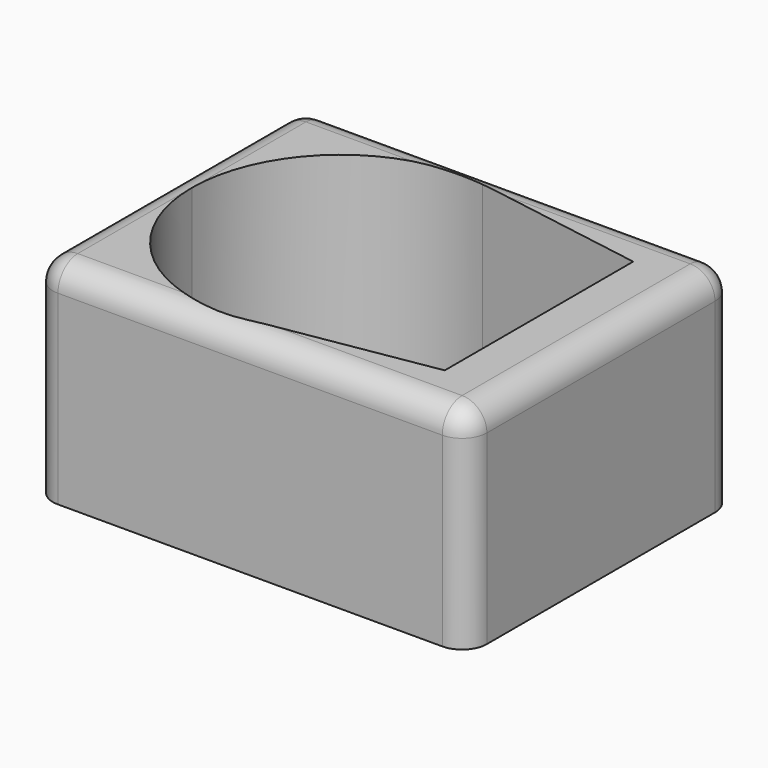
from build123d import *

# Parameters (mm, degrees)
F0_W         = 35
F0_H         = 27
F1_DEPTH     = 15
F2_DEPTH     = 2
F3_T1_DEPTH  = 20
F3_T3_DEPTH  = 31
F3_T5_DEPTH  = 23
F3_S9_W      = 2
F3_S9_H      = 2
F3_T10_DEPTH = 2
F3_S15_W     = 2
F3_S15_H     = 2
F3_T16_DEPTH = 2
F3_S21_W     = 2
F3_S21_H     = 2
F3_T22_DEPTH = 2
F3_S27_W     = 2
F3_S27_H     = 2
F3_T28_DEPTH = 2


# Not quite as in the source:
# - a fillet or chamfer that OpenCascade refuses, or shapes differently, is made with other operations: its cross-section is extruded or revolved along the edge and cut away or added


with BuildPart() as f1:
    # F0 (on Top) → F1 (new body)
    with BuildSketch(Plane.XY):
        with Locations((-13.2022674233, 7.6325895488)):
            Rectangle(F0_W, F0_H)
        with BuildLine():
            Line((-14.73041686, 19.4694728107), (-0.7022674233, 17.1325895488))
            Line((-0.7022674233, 17.1325895488), (-0.7022674233, 7.6325895488))
            Line((-0.7022674233, 7.6325895488), (-0.7022674233, -1.8674104512))
            Line((-0.7022674233, -1.8674104512), (-14.73041686, -4.2042937131))
            ThreePointArc((-14.73041686, -4.2042937131), (-24.4591286842, -1.5233431387), (-28.7022674233, 7.6325895488))
            ThreePointArc((-28.7022674233, 7.6325895488), (-24.4591286842, 16.7885222364), (-14.73041686, 19.4694728107))
        make_face(mode=Mode.SUBTRACT)
    extrude(amount=F1_DEPTH)

    # F0 (on Top) → F2 (join)
    with BuildSketch(Plane.XY):
        with Locations((-13.2022674233, 7.6325895488)):
            Rectangle(F0_W, F0_H)
        with BuildLine():
            Line((-14.73041686, 19.4694728107), (-0.7022674233, 17.1325895488))
            Line((-0.7022674233, 17.1325895488), (-0.7022674233, 7.6325895488))
            Line((-0.7022674233, 7.6325895488), (-0.7022674233, -1.8674104512))
            Line((-0.7022674233, -1.8674104512), (-14.73041686, -4.2042937131))
            ThreePointArc((-14.73041686, -4.2042937131), (-24.4591286842, -1.5233431387), (-28.7022674233, 7.6325895488))
            ThreePointArc((-28.7022674233, 7.6325895488), (-24.4591286842, 16.7885222364), (-14.73041686, 19.4694728107))
        make_face(mode=Mode.SUBTRACT)
        with BuildLine():
            ThreePointArc((-14.73041686, -4.2042937131), (-7.5463347357, -0.1242717121), (-4.7022674233, 7.6325895488))
            Line((-4.7022674233, 7.6325895488), (-28.7022674233, 7.6325895488))
            ThreePointArc((-28.7022674233, 7.6325895488), (-24.4591286842, -1.5233431387), (-14.73041686, -4.2042937131))
        make_face()
        with BuildLine():
            ThreePointArc((-4.7022674233, 7.6325895488), (-7.5463347357, 15.3894508097), (-14.73041686, 19.4694728107))
            ThreePointArc((-14.73041686, 19.4694728107), (-24.4591286842, 16.7885222364), (-28.7022674233, 7.6325895488))
            Line((-28.7022674233, 7.6325895488), (-4.7022674233, 7.6325895488))
        make_face()
        with BuildLine():
            Line((-0.7022674233, 7.6325895488), (-0.7022674233, 17.1325895488))
            Line((-0.7022674233, 17.1325895488), (-14.73041686, 19.4694728107))
            ThreePointArc((-14.73041686, 19.4694728107), (-7.5463347357, 15.3894508097), (-4.7022674233, 7.6325895488))
            Line((-4.7022674233, 7.6325895488), (-0.7022674233, 7.6325895488))
        make_face()
        with BuildLine():
            Line((-0.7022674233, -1.8674104512), (-0.7022674233, 7.6325895488))
            Line((-0.7022674233, 7.6325895488), (-4.7022674233, 7.6325895488))
            ThreePointArc((-4.7022674233, 7.6325895488), (-7.5463347357, -0.1242717121), (-14.73041686, -4.2042937131))
            Line((-14.73041686, -4.2042937131), (-0.7022674233, -1.8674104512))
        make_face()
    extrude(amount=-F2_DEPTH)

    # F3: fillet of radius 2 on 8 edges, made by hand

    # F3_s2 → F3_t1 (cut)
    with BuildSketch(Plane.XY.offset(-7)):
        with BuildLine():
            ThreePointArc((-30.7022674233, -3.8674104512), (-30.1164809856, -5.2816240135), (-28.7022674233, -5.8674104512))
            Line((-28.7022674233, -5.8674104512), (-30.7022674233, -5.8674104512))
            Line((-30.7022674233, -5.8674104512), (-30.7022674233, -3.8674104512))
        make_face()
        with BuildLine():
            ThreePointArc((4.2977325767, -3.8674104512), (3.7119461391, -5.2816240135), (2.2977325767, -5.8674104512))
            Line((2.2977325767, -5.8674104512), (4.2977325767, -5.8674104512))
            Line((4.2977325767, -5.8674104512), (4.2977325767, -3.8674104512))
        make_face()
        with BuildLine():
            ThreePointArc((4.2977325767, 19.1325895488), (3.7119461391, 20.5468031112), (2.2977325767, 21.1325895488))
            Line((2.2977325767, 21.1325895488), (4.2977325767, 21.1325895488))
            Line((4.2977325767, 21.1325895488), (4.2977325767, 19.1325895488))
        make_face()
        with BuildLine():
            ThreePointArc((-30.7022674233, 19.1325895488), (-30.1164809856, 20.5468031112), (-28.7022674233, 21.1325895488))
            Line((-28.7022674233, 21.1325895488), (-30.7022674233, 21.1325895488))
            Line((-30.7022674233, 21.1325895488), (-30.7022674233, 19.1325895488))
        make_face()
    extrude(amount=F3_T1_DEPTH, mode=Mode.SUBTRACT)

    # F3_s4 → F3_t3 (cut)
    with BuildSketch(Plane.YZ.offset(-28.7022674233)):
        with BuildLine():
            ThreePointArc((-3.8674104512, 15), (-5.2816240135, 14.4142135624), (-5.8674104512, 13))
            Line((-5.8674104512, 13), (-5.8674104512, 15))
            Line((-5.8674104512, 15), (-3.8674104512, 15))
        make_face()
        with BuildLine():
            ThreePointArc((21.1325895488, 13), (20.5468031112, 14.4142135624), (19.1325895488, 15))
            Line((19.1325895488, 15), (21.1325895488, 15))
            Line((21.1325895488, 15), (21.1325895488, 13))
        make_face()
    extrude(amount=F3_T3_DEPTH, mode=Mode.SUBTRACT)

    # F3_s6 → F3_t5 (cut)
    with BuildSketch(Plane.XZ.offset(-19.1325895488)):
        with BuildLine():
            ThreePointArc((4.2977325767, 13), (3.7119461391, 14.4142135624), (2.2977325767, 15))
            Line((2.2977325767, 15), (4.2977325767, 15))
            Line((4.2977325767, 15), (4.2977325767, 13))
        make_face()
        with BuildLine():
            ThreePointArc((-30.7022674233, 13), (-30.1164809856, 14.4142135624), (-28.7022674233, 15))
            Line((-28.7022674233, 15), (-30.7022674233, 15))
            Line((-30.7022674233, 15), (-30.7022674233, 13))
        make_face()
    extrude(amount=F3_T5_DEPTH, mode=Mode.SUBTRACT)


with BuildPart() as f3_tool8:
    # F3_s9 → F3_t10 (new body)
    with BuildSketch(Plane.YZ.offset(-28.7022674233)):
        with Locations((-4.8674104512, 14)):
            Rectangle(F3_S9_W, F3_S9_H)
    extrude(amount=-F3_T10_DEPTH)

    # F3_s11 → F3_t12 (revolve, cut)
    with BuildSketch(Plane(origin=(-28.7022674233, -3.8674104512, 13), x_dir=(0, 0.7071067812, -0.7071067812), z_dir=(0, 0.7071067812, 0.7071067812))):
        with BuildLine():
            ThreePointArc((0, -2), (2, 0), (0, 2))
            Line((0, 2), (0, -2))
        make_face()
    revolve(axis=Axis((-28.7022674233, -3.8674104512, 13), (-1, 0, 0)), mode=Mode.SUBTRACT)


with BuildPart() as f1_1:
    add(f1.part)

    # F3_t7: cut F3_tool8
    add(f3_tool8.part, mode=Mode.SUBTRACT)


with BuildPart() as f3_tool14:
    # F3_s15 → F3_t16 (new body)
    with BuildSketch(Plane.YZ.offset(2.2977325767)):
        with Locations((-4.8674104512, 14)):
            Rectangle(F3_S15_W, F3_S15_H)
    extrude(amount=F3_T16_DEPTH)

    # F3_s17 → F3_t18 (revolve, cut)
    with BuildSketch(Plane(origin=(2.2977325767, -3.8674104512, 13), x_dir=(0, 0.7071067812, -0.7071067812), z_dir=(0, -0.7071067812, -0.7071067812))):
        with BuildLine():
            ThreePointArc((0, -2), (2, 0), (0, 2))
            Line((0, 2), (0, -2))
        make_face()
    revolve(axis=Axis((2.2977325767, -3.8674104512, 13), (1, 0, 0)), mode=Mode.SUBTRACT)


with BuildPart() as f1_2:
    add(f1_1.part)

    # F3_t13: cut F3_tool14
    add(f3_tool14.part, mode=Mode.SUBTRACT)


with BuildPart() as f3_tool20:
    # F3_s21 → F3_t22 (new body)
    with BuildSketch(Plane.YZ.offset(2.2977325767)):
        with Locations((20.1325895488, 14)):
            Rectangle(F3_S21_W, F3_S21_H)
    extrude(amount=F3_T22_DEPTH)

    # F3_s23 → F3_t24 (revolve, cut)
    with BuildSketch(Plane(origin=(2.2977325767, 19.1325895488, 13), x_dir=(0, -0.7071067812, -0.7071067812), z_dir=(0, -0.7071067812, 0.7071067812))):
        with BuildLine():
            ThreePointArc((0, -2), (2, 0), (0, 2))
            Line((0, 2), (0, -2))
        make_face()
    revolve(axis=Axis((2.2977325767, 19.1325895488, 13), (1, 0, 0)), mode=Mode.SUBTRACT)


with BuildPart() as f1_3:
    add(f1_2.part)

    # F3_t19: cut F3_tool20
    add(f3_tool20.part, mode=Mode.SUBTRACT)


with BuildPart() as f3_tool26:
    # F3_s27 → F3_t28 (new body)
    with BuildSketch(Plane.YZ.offset(-28.7022674233)):
        with Locations((20.1325895488, 14)):
            Rectangle(F3_S27_W, F3_S27_H)
    extrude(amount=-F3_T28_DEPTH)

    # F3_s29 → F3_t30 (revolve, cut)
    with BuildSketch(Plane(origin=(-28.7022674233, 19.1325895488, 13), x_dir=(0, -0.7071067812, -0.7071067812), z_dir=(0, 0.7071067812, -0.7071067812))):
        with BuildLine():
            ThreePointArc((0, -2), (2, 0), (0, 2))
            Line((0, 2), (0, -2))
        make_face()
    revolve(axis=Axis((-28.7022674233, 19.1325895488, 13), (-1, 0, 0)), mode=Mode.SUBTRACT)


with BuildPart() as f1_4:
    add(f1_3.part)

    # F3_t25: cut F3_tool26
    add(f3_tool26.part, mode=Mode.SUBTRACT)


solid = f1_4.part
